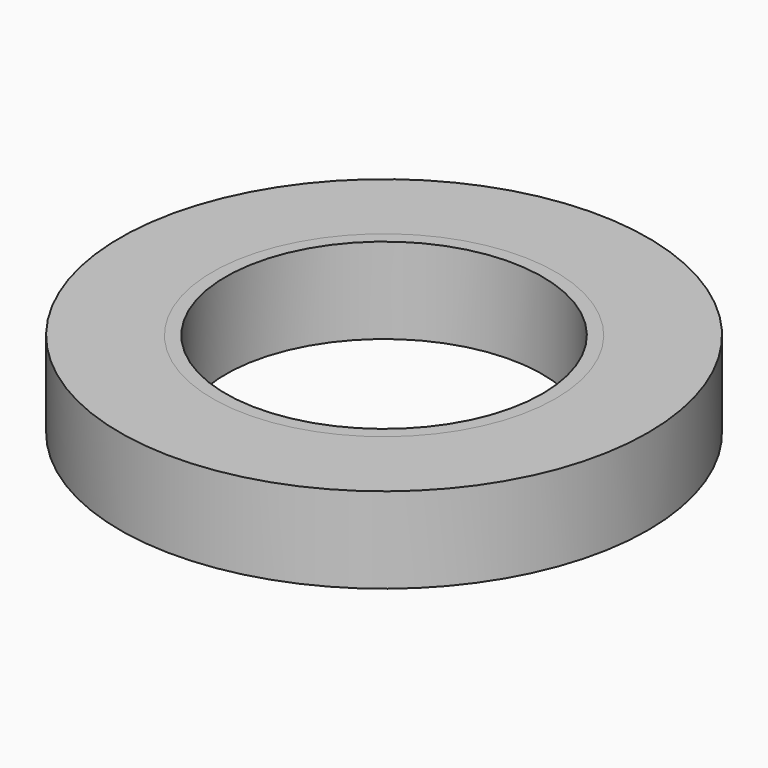
from build123d import *

# Parameters (mm, degrees)
F0_R     = 41.275
F0_R_2   = 38.1
F1_DEPTH = 20.6375
F2_R     = 63.5
F2_R_2   = 41.275
F3_DEPTH = 20.6375


# Not quite as in the source:
# - a length typed as a fraction of an inch, garbled in the dataset ("3 / 203.2 mm" for 3/8 in), is restored


with BuildPart() as f1:
    # F0 (on Top) → F1 (new body)
    with BuildSketch(Plane.XY):
        Circle(F0_R)
        Circle(F0_R_2, mode=Mode.SUBTRACT)
    extrude(amount=F1_DEPTH)


with BuildPart() as f3:
    # F2 (on Top) → F3 (new body)
    with BuildSketch(Plane.XY):
        Circle(F2_R)
        Circle(F2_R_2, mode=Mode.SUBTRACT)
    extrude(amount=F3_DEPTH)


solid = Compound([f1.part, f3.part])
